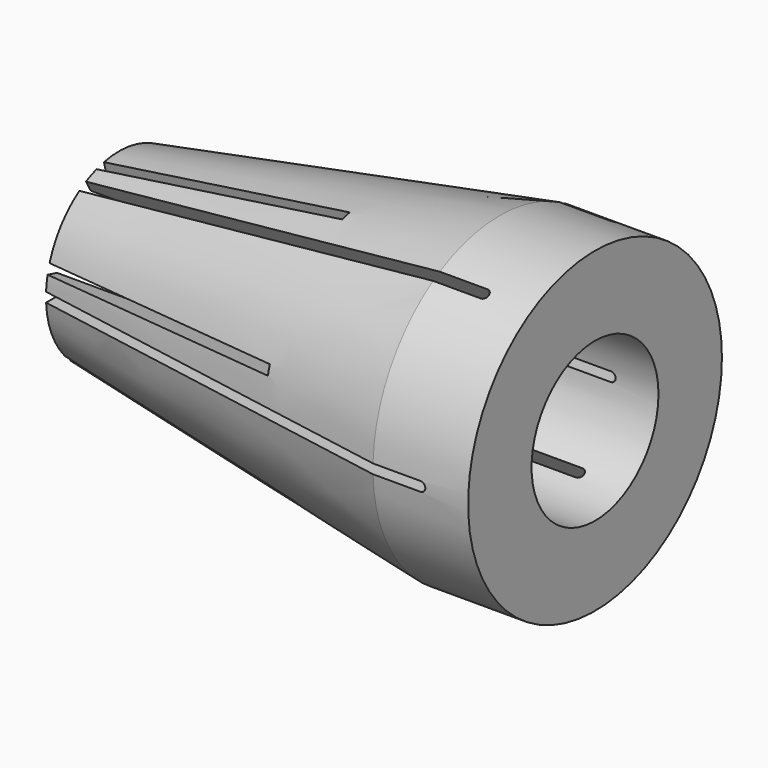
from build123d import *

# Parameters (mm, degrees)
F2_R            = 3.175
F3_DEPTH        = 19.051
F5_DEPTH        = 6.351
F5_COPIES_COUNT = 6
F8_W            = 10.2112228051
F8_H            = 0.381
F9_DEPTH        = 8.9812562625
F9_COPIES_COUNT = 6


# Not quite as in the source:
# - a pattern or mirror of a feature is missing from the dataset's text; its kind, count and spacing are read off the source's solid


with BuildPart() as f1:
    # F0 (on Top) → F1 (revolve)
    with BuildSketch(Plane.XY):
        Polygon((0, 3.662776814), (0, 0), (19.05, 0), (19.05, 6.35), (15.24, 6.35), align=None)
    revolve(axis=Axis((9.525, 0, 0), (1, 0, 0)))

    # F2 (on face) → F3 (cut, through all)
    with BuildSketch(Plane.YZ.offset(19.05)):
        Circle(F2_R)
    extrude(amount=-F3_DEPTH, mode=Mode.SUBTRACT)

    # F4 (on Front) → F5 (cut, through all)
    with BuildSketch(Plane.XZ):
        with BuildLine():
            Line((0, 0.1905), (0, -0.1905))
            Line((0, -0.1905), (17.145, -0.1905))
            ThreePointArc((17.145, -0.1905), (17.2797038418, -0.1347038418), (17.3355, 0))
            ThreePointArc((17.3355, 0), (17.2797038418, 0.1347038418), (17.145, 0.1905))
            Line((17.145, 0.1905), (0, 0.1905))
        make_face()
    f5 = extrude(amount=-F5_DEPTH, mode=Mode.SUBTRACT)

    # F5_copies: F5 ×6 about axis
    f5_copies_axis = Axis((0, 0, 0), (1, 0, 0))
    for i in range(1, F5_COPIES_COUNT):
        add(f5.rotate(f5_copies_axis, i * 360 / F5_COPIES_COUNT), mode=Mode.SUBTRACT)

    # F8 (on face) → F9 (cut, through all)
    with BuildSketch(Plane(origin=(0, 0, 0), x_dir=(-1, 0, 0), z_dir=(0, 0.7071067812, 0.7071067812))):
        with Locations((-5.1056114025, 0)):
            Rectangle(F8_W, F8_H)
    f9 = extrude(amount=-F9_DEPTH, mode=Mode.SUBTRACT)

    # F9_copies: F9 ×6 about axis
    f9_copies_axis = Axis((0, 0, 0), (1, 0, 0))
    for i in range(1, F9_COPIES_COUNT):
        add(f9.rotate(f9_copies_axis, i * 360 / F9_COPIES_COUNT), mode=Mode.SUBTRACT)


solid = f1.part
